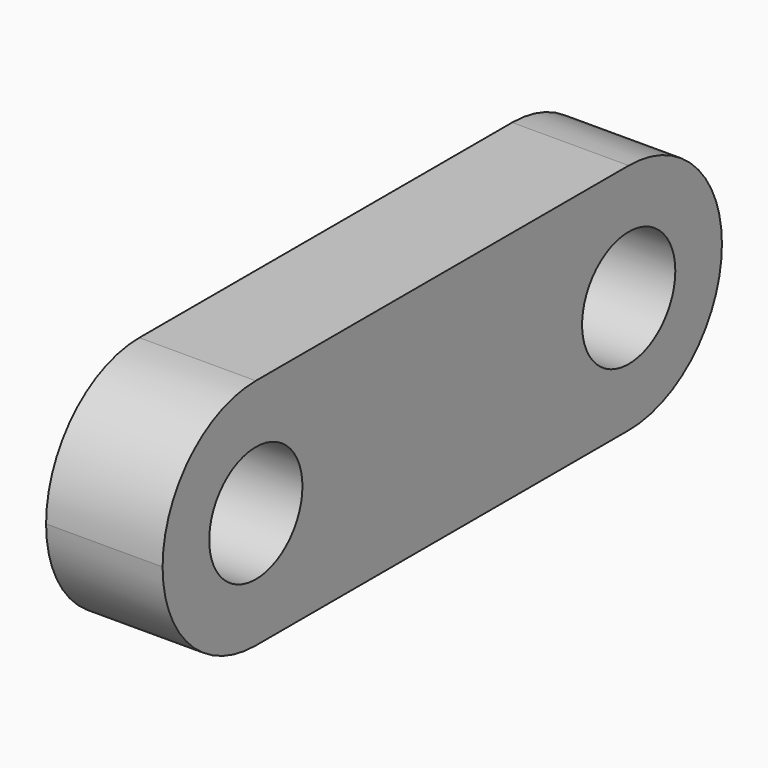
from build123d import *

# Parameters (mm, degrees)
F0_W     = 300
F0_H     = 100
F1_DEPTH = 50
F2_R     = 49.99999
F3_R     = 25
F4_DEPTH = 50


# Not quite as in the source:
# - a fillet or chamfer is up to 0.001 mm smaller than in the source, because OpenCascade refuses the exact size


with BuildPart() as f1:
    # F0 (on Right) → F1 (new body)
    with BuildSketch(Plane.YZ):
        Rectangle(F0_W, F0_H)
    extrude(amount=F1_DEPTH)

    # F2 (radius 50 in the source; OpenCascade refuses exactly that, so slightly less here)
    f2_edges = [f1.edges().sort_by_distance(p)[0] for p in [
        (25, -150, 50),
        (25, -150, -50),
        (25, 150, 50),
        (25, 150, -50),
    ]]
    fillet(f2_edges, radius=F2_R)

    # F3 (on face) → F4 (cut)
    with BuildSketch(Plane.YZ.offset(50)):
        with Locations((-100, 0)):
            Circle(F3_R)
        with Locations((100, 0)):
            Circle(F3_R)
    extrude(amount=-F4_DEPTH, mode=Mode.SUBTRACT)


solid = f1.part
